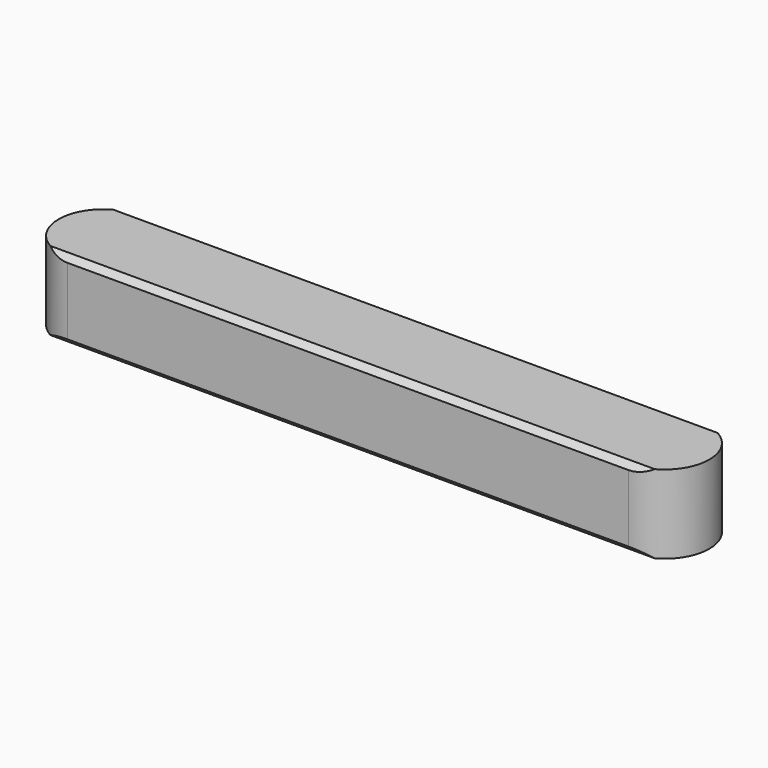
from build123d import *

# Parameters (mm, degrees)
F1_DEPTH    = 7
F2_T1_DEPTH = 54.3718610795


# Not quite as in the source:
# - a fillet or chamfer that OpenCascade refuses, or shapes differently, is made with other operations: its cross-section is extruded or revolved along the edge and cut away or added


with BuildPart() as f1:
    # F0 (on Top) → F1 (new body)
    with BuildSketch(Plane.XY):
        with BuildLine():
            Line((-25, -4), (25, -4))
            ThreePointArc((25, -4), (29, 0), (25, 4))
            Line((25, 4), (-25, 4))
            ThreePointArc((-25, 4), (-29, 0), (-25, -4))
        make_face()
    extrude(amount=F1_DEPTH)

    # F2: chamfer of 0.5 on 4 edges, made by hand

    # F2_s2 → F2_t1 (cut)
    with BuildSketch(Plane.YZ.offset(-27.1859305398)):
        Polygon((-4, 6.5), (-3.5, 7), (-4, 7), align=None)
        Polygon((4, 6.5), (3.5, 7), (4, 7), align=None)
        Polygon((-4, 0.5), (-3.5, 0), (-4, 0), align=None)
        Polygon((4, 0.5), (3.5, 0), (4, 0), align=None)
    extrude(amount=F2_T1_DEPTH, mode=Mode.SUBTRACT)


solid = f1.part
